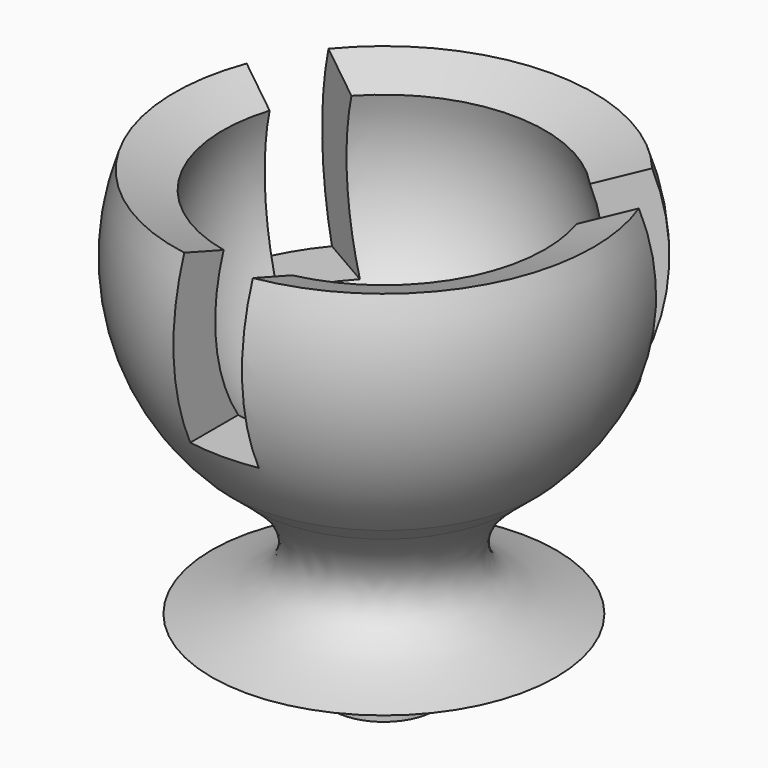
from build123d import *

# Parameters (mm, degrees)
F1_W            = 1.27
F1_H            = 6.35
F3_DEPTH        = 25.4
F3_COPIES_COUNT = 3


# Not quite as in the source:
# - a pattern or mirror of a feature is missing from the dataset's text; its kind, count and spacing are read off the source's solid


with BuildPart() as f2:
    # F0 (on Front) → F2 (revolve)
    with BuildSketch(Plane.XZ):
        with BuildLine():
            ThreePointArc((0, 1.7563040945), (2.5128555378, 2.1480616306), (4.7872059044, 3.286150964))
            add(Edge.make_bspline(
                [(5.7211114804, 4.0603454802), (5.4050531377, 3.7970740836), (5.0875138571, 3.5404942593), (4.7872059044, 3.286150964)],
                knots=[0, 0, 0, 0, 0.1185853602, 0.1185853602, 0.1185853602, 0.1185853602], degree=3))
            ThreePointArc((5.7211114804, 4.0603454802), (8.0413435548, 8.1453408488), (7.7571625846, 12.8346803777))
            Line((7.7571625846, 12.8346803777), (5.967048142, 12.1831320046))
            ThreePointArc((5.967048142, 12.1831320046), (5.2016154812, 6.3690937237), (0, 3.6613040945))
            Line((0, 3.6613040945), (0, 1.7563040945))
        make_face()
        with BuildLine():
            Line((1.9936987545, -1.6295855468), (6.3774073496, -1.6295855468))
            add(Edge.make_bspline(
                [(4.7872059044, 3.286150964), (4.1586216225, 2.7537767921), (3.0308358819, 1.6882127438), (2.8559446967, -0.3923291132), (4.7623664117, -1.1922165544), (6.3774073496, -1.6295855468)],
                knots=[0.1185853602, 0.1185853602, 0.1185853602, 0.1185853602, 0.3668002104, 0.6247109414, 1, 1, 1, 1], degree=3))
            ThreePointArc((4.7872059044, 3.286150964), (2.5128555378, 2.1480616306), (0, 1.7563040945))
            Line((0, 1.7563040945), (0, -1.6295855468))
            Line((0, -1.6295855468), (0.1668176933, -1.6295855468))
            Line((0.1668176933, -1.6295855468), (1.9936987545, -1.6295855468))
        make_face()
        Polygon((1.905, -4.1695855468), (1.9936987545, -1.6295855468), (0.1668176933, -1.6295855468), (0, -1.6295855468), (0, -4.1695855468), align=None)
    revolve(axis=Axis((0, 0, 5.9904144532), (0, 0, -1)))

    # F1 (on Front) → F3 (cut)
    with BuildSketch(Plane.XZ):
        with Locations((-0.635, 9.7055145408)):
            Rectangle(F1_W, F1_H)
        with Locations((0.635, 9.7055145408)):
            Rectangle(F1_W, F1_H)
    f3 = extrude(amount=F3_DEPTH, mode=Mode.SUBTRACT)

    # F3_copies: F3 ×3 about axis
    f3_copies_axis = Axis((0, 0, 0), (0, 0, 1))
    for i in range(1, F3_COPIES_COUNT):
        add(f3.rotate(f3_copies_axis, i * 360 / F3_COPIES_COUNT), mode=Mode.SUBTRACT)


solid = f2.part
